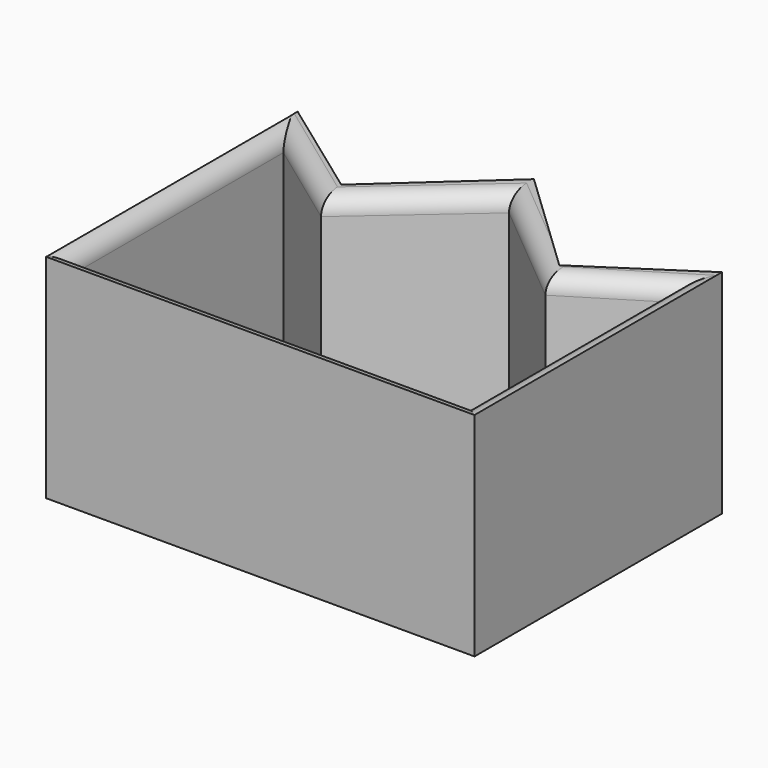
from build123d import *

# Parameters (mm, degrees)
F2_DEPTH     = 25
F3_T1_DEPTH  = 46.6258954257
F3_T6_DEPTH  = 35.914994888
F3_T11_DEPTH = 23.17796644
F3_T16_DEPTH = 27.2775423945
F3_T21_DEPTH = 26.7037330094
F3_T26_DEPTH = 21.9083744996
F3_T31_DEPTH = 35.0703225657
F3_T37_DEPTH = 51.6258954257
F3_T43_DEPTH = 40.914994888
F3_T52_DEPTH = 23.17796644
F3_T57_DEPTH = 35.914994888
F3_T66_DEPTH = 26.7037330094
F3_T71_DEPTH = 27.2775423945
F3_T79_DEPTH = 35.0703225657
F3_T84_DEPTH = 21.9083744996
F3_T92_DEPTH = 51.6258954257
F3_T98_DEPTH = 40.0703225657


# Not quite as in the source:
# - a fillet or chamfer that OpenCascade refuses, or shapes differently, is made with other operations: its cross-section is extruded or revolved along the edge and cut away or added


with BuildPart() as f2:
    # F0 (on Top) → F2 (new body)
    with BuildSketch(Plane.XY):
        Polygon((-25.346679613, 20.7659546286), (-25.346679613, 0), (-25.346679613, -16.2133686244), (25.0412952155, -16.2133686244), (25.0412952155, 0), (25.0412952155, 20.1551914215), (12.5206476077, 11.909885332), (0, 23.819770664), (-13.1314117461, 11.909885332), align=None)
        Polygon((-23.6552227288, -14.3550904468), (-23.6552227288, 16.5599044412), (-13.0123551935, 8.7889218703), (0, 20.1551914215), (12.8346113488, 9.4646606594), (22.9706726968, 15.715232119), (22.9706726968, -14.3550904468), align=None, mode=Mode.SUBTRACT)
    extrude(amount=F2_DEPTH)

    # F3: fillet of radius 2 on 7 edges, made by hand

    # F3_s2 → F3_t1 (cut)
    with BuildSketch(Plane.YZ.offset(-23.6552227288)):
        with BuildLine():
            ThreePointArc((-14.3550904468, 23), (-14.9408768844, 24.4142135624), (-16.3550904468, 25))
            Line((-16.3550904468, 25), (-14.3550904468, 25))
            Line((-14.3550904468, 25), (-14.3550904468, 23))
        make_face()
    extrude(amount=F3_T1_DEPTH, mode=Mode.SUBTRACT)


with BuildPart() as f3_tool4:
    # F3_s5 → F3_t6 (new body)
    with BuildSketch(Plane.XZ.offset(14.3550904468)):
        with BuildLine():
            ThreePointArc((-23.6552227288, 23), (-24.2410091665, 24.4142135624), (-25.6552227288, 25))
            Line((-25.6552227288, 25), (-23.6552227288, 25))
            Line((-23.6552227288, 25), (-23.6552227288, 23))
        make_face()
    extrude(amount=-F3_T6_DEPTH)

    split(bisect_by=Plane(origin=(-0.3391697192, -0.4645150547, 0), x_dir=(0, 0, 1), z_dir=(-0.5896951253, -0.8076259402, 0)), keep=Keep.TOP)


with BuildPart() as f2_1:
    add(f2.part)

    # F3_t3: cut F3_tool4
    add(f3_tool4.part, mode=Mode.SUBTRACT)


with BuildPart() as f3_tool9:
    # F3_s10 → F3_t11 (new body)
    with BuildSketch(Plane(origin=(-27.3541827104, 19.9728951224, 0), x_dir=(0, 0, 1), z_dir=(0.8076259402, -0.5896951253, 0))):
        with BuildLine():
            ThreePointArc((23, 0.5751611378), (24.4142135624, -0.0106252998), (25, -1.4248388622))
            Line((25, -1.4248388622), (25, 0.5751611378))
            Line((25, 0.5751611378), (23, 0.5751611378))
        make_face()
    extrude(amount=F3_T11_DEPTH)

    split(bisect_by=Plane.YZ.offset(-23.6552227288), keep=Keep.TOP)


with BuildPart() as f2_2:
    add(f2_1.part)

    # F3_t8: cut F3_tool9
    add(f3_tool9.part, mode=Mode.SUBTRACT)


with BuildPart() as f3_tool14:
    # F3_s15 → F3_t16 (new body)
    with BuildSketch(Plane(origin=(-6.7919181581, -5.9327286573, 0), x_dir=(0, 0, 1), z_dir=(0.7531369275, 0.6578637917, 0))):
        with BuildLine():
            ThreePointArc((23, -15.1796189401), (24.4142135624, -15.7654053777), (25, -17.1796189401))
            Line((25, -17.1796189401), (25, -15.1796189401))
            Line((25, -15.1796189401), (23, -15.1796189401))
        make_face()
    extrude(amount=F3_T16_DEPTH)

    split(bisect_by=Plane(origin=(9.9115559644, 11.8994062592, 0), x_dir=(0, 0, 1), z_dir=(-0.6400084793, -0.7683678458, 0)), keep=Keep.TOP)


with BuildPart() as f2_3:
    add(f2_2.part)

    # F3_t13: cut F3_tool14
    add(f3_tool14.part, mode=Mode.SUBTRACT)


with BuildPart() as f3_tool19:
    # F3_s20 → F3_t21 (new body)
    with BuildSketch(Plane(origin=(-13.7533951932, 11.4558275588, 0), x_dir=(0, 0, 1), z_dir=(0.7683678458, -0.6400084793, 0))):
        with BuildLine():
            ThreePointArc((23, -15.4866010137), (24.4142135624, -16.0723874513), (25, -17.4866010137))
            Line((25, -17.4866010137), (25, -15.4866010137))
            Line((25, -15.4866010137), (23, -15.4866010137))
        make_face()
    extrude(amount=F3_T21_DEPTH)

    split(bisect_by=Plane(origin=(-9.9861216728, 11.432331569, 0), x_dir=(0, 0, 1), z_dir=(0.6578637917, -0.7531369275, 0)), keep=Keep.TOP)


with BuildPart() as f2_4:
    add(f2_3.part)

    # F3_t18: cut F3_tool19
    add(f3_tool19.part, mode=Mode.SUBTRACT)


with BuildPart() as f3_tool24:
    # F3_s25 → F3_t26 (new body)
    with BuildSketch(Plane(origin=(9.271243063, 5.7172668253, 0), x_dir=(0, 0, 1), z_dir=(0.8511708587, 0.5248887209, 0))):
        with BuildLine():
            ThreePointArc((23, -1.3193006058), (24.4142135624, -1.9050870434), (25, -3.3193006058))
            Line((25, -3.3193006058), (25, -1.3193006058))
            Line((25, -1.3193006058), (23, -1.3193006058))
        make_face()
    extrude(amount=F3_T26_DEPTH)

    split(bisect_by=Plane.YZ.offset(22.9706726968), keep=Keep.BOTTOM)


with BuildPart() as f2_5:
    add(f2_4.part)

    # F3_t23: cut F3_tool24
    add(f3_tool24.part, mode=Mode.SUBTRACT)


with BuildPart() as f3_tool29:
    # F3_s30 → F3_t31 (new body)
    with BuildSketch(Plane.XZ.offset(-20.715232119)):
        with BuildLine():
            ThreePointArc((22.9706726968, 23), (23.5564591345, 24.4142135624), (24.9706726968, 25))
            Line((24.9706726968, 25), (22.9706726968, 25))
            Line((22.9706726968, 25), (22.9706726968, 23))
        make_face()
    extrude(amount=F3_T31_DEPTH)

    split(bisect_by=Plane(origin=(-0.6924860075, 1.1229502295, 0), x_dir=(0, 0, 1), z_dir=(0.5248887209, -0.8511708587, 0)), keep=Keep.TOP)


with BuildPart() as f2_6:
    add(f2_5.part)

    # F3_t28: cut F3_tool29
    add(f3_tool29.part, mode=Mode.SUBTRACT)


with BuildPart() as f3_tool35:
    # F3_s36 → F3_t37 (new body)
    with BuildSketch(Plane.YZ.offset(22.9706726968)):
        with BuildLine():
            ThreePointArc((-14.3550904468, 23), (-14.9408768844, 24.4142135624), (-16.3550904468, 25))
            Line((-16.3550904468, 25), (-14.3550904468, 25))
            Line((-14.3550904468, 25), (-14.3550904468, 23))
        make_face()
    extrude(amount=-F3_T37_DEPTH)

    split(bisect_by=Plane.YZ.offset(-25.346679613), keep=Keep.TOP)

    split(bisect_by=Plane.YZ.offset(-23.6552227288), keep=Keep.BOTTOM)

    split(bisect_by=Plane.XZ.offset(16.2133686244), keep=Keep.BOTTOM)


with BuildPart() as f3_tool41:
    # F3_s42 → F3_t43 (new body)
    with BuildSketch(Plane.XZ.offset(19.3550904468)):
        with BuildLine():
            ThreePointArc((-23.6552227288, 23), (-24.2410091665, 24.4142135624), (-25.6552227288, 25))
            Line((-25.6552227288, 25), (-23.6552227288, 25))
            Line((-23.6552227288, 25), (-23.6552227288, 23))
        make_face()
    extrude(amount=-F3_T43_DEPTH)

    split(bisect_by=Plane.YZ.offset(-25.346679613), keep=Keep.TOP)

    split(bisect_by=Plane.XZ.offset(14.3550904468), keep=Keep.TOP)

    split(bisect_by=Plane.XZ.offset(16.2133686244), keep=Keep.BOTTOM)


with BuildPart() as f3_tool35_1:
    add(f3_tool35.part)

    # F3_t47: intersect F3_tool41
    add(f3_tool41.part, mode=Mode.INTERSECT)


with BuildPart() as f2_7:
    add(f2_6.part)

    # F3_t33: cut F3_tool35
    add(f3_tool35_1.part, mode=Mode.SUBTRACT)


with BuildPart() as f3_tool50:
    # F3_s51 → F3_t52 (new body)
    with BuildSketch(Plane(origin=(-27.3541827104, 19.9728951224, 0), x_dir=(0, 0, 1), z_dir=(0.8076259402, -0.5896951253, 0))):
        with BuildLine():
            ThreePointArc((23, 0.5751611378), (24.4142135624, -0.0106252998), (25, -1.4248388622))
            Line((25, -1.4248388622), (25, 0.5751611378))
            Line((25, 0.5751611378), (23, 0.5751611378))
        make_face()
    extrude(amount=F3_T52_DEPTH)

    split(bisect_by=Plane.YZ.offset(-25.346679613), keep=Keep.TOP)

    split(bisect_by=Plane.YZ.offset(-23.6552227288), keep=Keep.BOTTOM)


with BuildPart() as f3_tool55:
    # F3_s56 → F3_t57 (new body)
    with BuildSketch(Plane.XZ.offset(14.3550904468)):
        with BuildLine():
            ThreePointArc((-23.6552227288, 23), (-24.2410091665, 24.4142135624), (-25.6552227288, 25))
            Line((-25.6552227288, 25), (-23.6552227288, 25))
            Line((-23.6552227288, 25), (-23.6552227288, 23))
        make_face()
    extrude(amount=-F3_T57_DEPTH)

    split(bisect_by=Plane.YZ.offset(-25.346679613), keep=Keep.TOP)

    split(bisect_by=Plane(origin=(-0.3391697192, -0.4645150547, 0), x_dir=(0, 0, 1), z_dir=(0.5896951253, 0.8076259402, 0)), keep=Keep.TOP)

    split(bisect_by=Plane(origin=(1.1355795164, 1.5663165579, 0), x_dir=(0, 0, 1), z_dir=(-0.5869675755, -0.8096104405, 0)), keep=Keep.TOP)


with BuildPart() as f3_tool50_1:
    add(f3_tool50.part)

    # F3_t61: intersect F3_tool55
    add(f3_tool55.part, mode=Mode.INTERSECT)


with BuildPart() as f2_8:
    add(f2_7.part)

    # F3_t48: cut F3_tool50
    add(f3_tool50_1.part, mode=Mode.SUBTRACT)


with BuildPart() as f3_tool64:
    # F3_s65 → F3_t66 (new body)
    with BuildSketch(Plane(origin=(-13.7533951932, 11.4558275588, 0), x_dir=(0, 0, 1), z_dir=(0.7683678458, -0.6400084793, 0))):
        with BuildLine():
            ThreePointArc((23, -15.4866010137), (24.4142135624, -16.0723874513), (25, -17.4866010137))
            Line((25, -17.4866010137), (25, -15.4866010137))
            Line((25, -15.4866010137), (23, -15.4866010137))
        make_face()
    extrude(amount=F3_T66_DEPTH)

    split(bisect_by=Plane(origin=(-9.9861216728, 11.432331569, 0), x_dir=(0, 0, 1), z_dir=(-0.6578637917, 0.7531369275, 0)), keep=Keep.TOP)

    split(bisect_by=Plane(origin=(-11.8533399075, 13.0690667923, 0), x_dir=(0, 0, 1), z_dir=(0.6718149465, -0.7407190274, 0)), keep=Keep.TOP)


with BuildPart() as f3_tool69:
    # F3_s70 → F3_t71 (new body)
    with BuildSketch(Plane(origin=(-6.7919181581, -5.9327286573, 0), x_dir=(0, 0, 1), z_dir=(0.7531369275, 0.6578637917, 0))):
        with BuildLine():
            ThreePointArc((23, -15.1796189401), (24.4142135624, -15.7654053777), (25, -17.1796189401))
            Line((25, -17.1796189401), (25, -15.1796189401))
            Line((25, -15.1796189401), (23, -15.1796189401))
        make_face()
    extrude(amount=F3_T71_DEPTH)

    split(bisect_by=Plane(origin=(9.9115559644, 11.8994062592, 0), x_dir=(0, 0, 1), z_dir=(0.6400084793, 0.7683678458, 0)), keep=Keep.TOP)

    split(bisect_by=Plane(origin=(11.8950073251, 12.5050066275, 0), x_dir=(0, 0, 1), z_dir=(-0.6892137971, -0.7245580322, 0)), keep=Keep.TOP)


with BuildPart() as f3_tool64_1:
    add(f3_tool64.part)

    # F3_t74: intersect F3_tool69
    add(f3_tool69.part, mode=Mode.INTERSECT)


with BuildPart() as f2_9:
    add(f2_8.part)

    # F3_t62: cut F3_tool64
    add(f3_tool64_1.part, mode=Mode.SUBTRACT)


with BuildPart() as f3_tool77:
    # F3_s78 → F3_t79 (new body)
    with BuildSketch(Plane.XZ.offset(-20.715232119)):
        with BuildLine():
            ThreePointArc((22.9706726968, 23), (23.5564591345, 24.4142135624), (24.9706726968, 25))
            Line((24.9706726968, 25), (22.9706726968, 25))
            Line((22.9706726968, 25), (22.9706726968, 23))
        make_face()
    extrude(amount=F3_T79_DEPTH)

    split(bisect_by=Plane(origin=(-0.6924860075, 1.1229502295, 0), x_dir=(0, 0, 1), z_dir=(-0.5248887209, 0.8511708587, 0)), keep=Keep.TOP)

    split(bisect_by=Plane(origin=(-1.6832736623, 2.556081742, 0), x_dir=(0, 0, 1), z_dir=(0.5499906424, -0.8351708168, 0)), keep=Keep.TOP)


with BuildPart() as f3_tool82:
    # F3_s83 → F3_t84 (new body)
    with BuildSketch(Plane(origin=(9.271243063, 5.7172668253, 0), x_dir=(0, 0, 1), z_dir=(0.8511708587, 0.5248887209, 0))):
        with BuildLine():
            ThreePointArc((23, -1.3193006058), (24.4142135624, -1.9050870434), (25, -3.3193006058))
            Line((25, -3.3193006058), (25, -1.3193006058))
            Line((25, -1.3193006058), (23, -1.3193006058))
        make_face()
    extrude(amount=F3_T84_DEPTH)

    split(bisect_by=Plane.YZ.offset(22.9706726968), keep=Keep.TOP)

    split(bisect_by=Plane.YZ.offset(25.0412952155), keep=Keep.BOTTOM)


with BuildPart() as f3_tool77_1:
    add(f3_tool77.part)

    # F3_t87: intersect F3_tool82
    add(f3_tool82.part, mode=Mode.INTERSECT)


with BuildPart() as f2_10:
    add(f2_9.part)

    # F3_t75: cut F3_tool77
    add(f3_tool77_1.part, mode=Mode.SUBTRACT)


with BuildPart() as f3_tool90:
    # F3_s91 → F3_t92 (new body)
    with BuildSketch(Plane.YZ.offset(27.9706726968)):
        with BuildLine():
            ThreePointArc((-14.3550904468, 23), (-14.9408768844, 24.4142135624), (-16.3550904468, 25))
            Line((-16.3550904468, 25), (-14.3550904468, 25))
            Line((-14.3550904468, 25), (-14.3550904468, 23))
        make_face()
    extrude(amount=-F3_T92_DEPTH)

    split(bisect_by=Plane.YZ.offset(22.9706726968), keep=Keep.TOP)

    split(bisect_by=Plane.YZ.offset(25.0412952155), keep=Keep.BOTTOM)

    split(bisect_by=Plane.XZ.offset(16.2133686244), keep=Keep.BOTTOM)


with BuildPart() as f3_tool96:
    # F3_s97 → F3_t98 (new body)
    with BuildSketch(Plane.XZ.offset(-20.715232119)):
        with BuildLine():
            ThreePointArc((22.9706726968, 23), (23.5564591345, 24.4142135624), (24.9706726968, 25))
            Line((24.9706726968, 25), (22.9706726968, 25))
            Line((22.9706726968, 25), (22.9706726968, 23))
        make_face()
    extrude(amount=F3_T98_DEPTH)

    split(bisect_by=Plane.XZ.offset(14.3550904468), keep=Keep.TOP)

    split(bisect_by=Plane.XZ.offset(16.2133686244), keep=Keep.BOTTOM)


with BuildPart() as f3_tool90_1:
    add(f3_tool90.part)

    # F3_t101: intersect F3_tool96
    add(f3_tool96.part, mode=Mode.INTERSECT)


with BuildPart() as f2_11:
    add(f2_10.part)

    # F3_t88: cut F3_tool90
    add(f3_tool90_1.part, mode=Mode.SUBTRACT)


solid = f2_11.part
